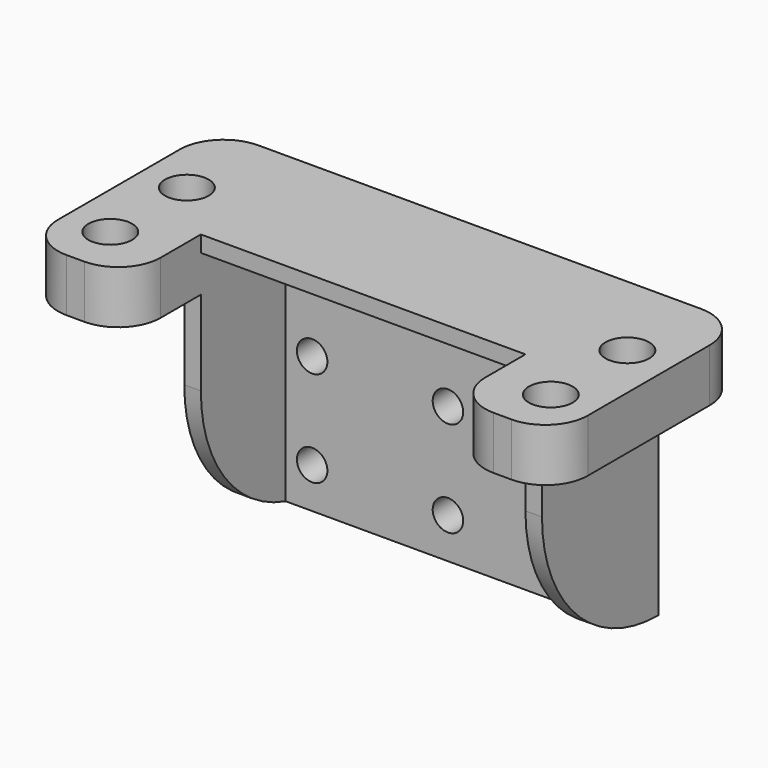
from build123d import *

# Parameters (mm, degrees)
F0_W          = 27
F0_H          = 21.4
F1_DEPTH      = 3
F2_R          = 1.15
F3_DEPTH      = 3.001
F5_DEPTH      = 8
F5_DEPTH_BACK = 3
F6_W          = 7.75
F6_H          = 4
F7_DEPTH      = 7
F8_R          = 1.65
F9_DEPTH      = 25
F10_F1_R      = 10.9999
F11_R         = 3.3
F12_R         = 3.2


# Not quite as in the source:
# - a fillet or chamfer is up to 0.001 mm smaller than in the source, because OpenCascade refuses the exact size


with BuildPart() as f1:
    # F0 (on Front) → F1 (new body)
    with BuildSketch(Plane.XZ):
        Rectangle(F0_W, F0_H)
    extrude(amount=-F1_DEPTH)

    # F2 (on Front) → F3 (cut, through all)
    with BuildSketch(Plane.XZ):
        with Locations((0, 7.225)):
            Circle(F2_R)
        Circle(F2_R)
        with Locations((0, -7.225)):
            Circle(F2_R)
        with Locations((10.25, 0)):
            Circle(F2_R)
        with Locations((10.25, 7.225)):
            Circle(F2_R)
        with Locations((10.25, -7.225)):
            Circle(F2_R)
        with Locations((-10.25, -7.225)):
            Circle(F2_R)
        with Locations((-10.25, 0)):
            Circle(F2_R)
        with Locations((-10.25, 7.225)):
            Circle(F2_R)
    extrude(amount=-F3_DEPTH, mode=Mode.SUBTRACT)

    # F4 (on Front) → F5 (join, two sides)
    with BuildSketch(Plane.XZ) as f5_sk:
        Polygon((20, 10.7), (0, 10.7), (-20, 10.7), (-20, 6.7), (-13.5, 6.7), (-13.5, -10.7), (-12.25, -10.7), (-12.25, 9.475), (0, 9.475), (12.25, 9.475), (12.25, -10.7), (13.5, -10.7), (13.5, 6.7), (20, 6.7), align=None)
    extrude(amount=F5_DEPTH)
    extrude(f5_sk.sketch, amount=-F5_DEPTH_BACK)

    # F6 (on face) → F7 (join)
    with BuildSketch(Plane.XZ.offset(8)):
        with Locations((16.125, 8.7)):
            Rectangle(F6_W, F6_H)
        with Locations((-16.125, 8.7)):
            Rectangle(F6_W, F6_H)
    extrude(amount=F7_DEPTH)

    # F8 (on face) → F9 (cut)
    with BuildSketch(Plane(origin=(0, 0, 6.7), x_dir=(1, 0, 0), z_dir=(0, 0, -1))):
        with Locations((-16.625, 3.85)):
            Circle(F8_R)
        with Locations((16.625, 3.85)):
            Circle(F8_R)
        with Locations((16.625, 11.075)):
            Circle(F8_R)
        with Locations((-16.625, 11.075)):
            Circle(F8_R)
    extrude(amount=-F9_DEPTH, mode=Mode.SUBTRACT)

    # F10: fillet of radius 11 on 2 edges, made by hand

    # F10_f1 (radius 11 in the source; OpenCascade refuses exactly that, so slightly less here)
    f10_f1_edges = [f1.edges().sort_by_distance(p)[0] for p in [
        (12.875, -8, -10.7),
    ]]
    fillet(f10_f1_edges, radius=F10_F1_R)

    # F11
    f11_edges = [f1.edges().sort_by_distance(p)[0] for p in [
        (20, 3, 8.7),
        (-20, 3, 8.7),
    ]]
    fillet(f11_edges, radius=F11_R)

    # F12
    f12_edges = [f1.edges().sort_by_distance(p)[0] for p in [
        (20, -15, 8.7),
        (12.25, -15, 8.7),
        (-12.25, -15, 8.7),
        (-20, -15, 8.7),
    ]]
    fillet(f12_edges, radius=F12_R)


solid = f1.part
